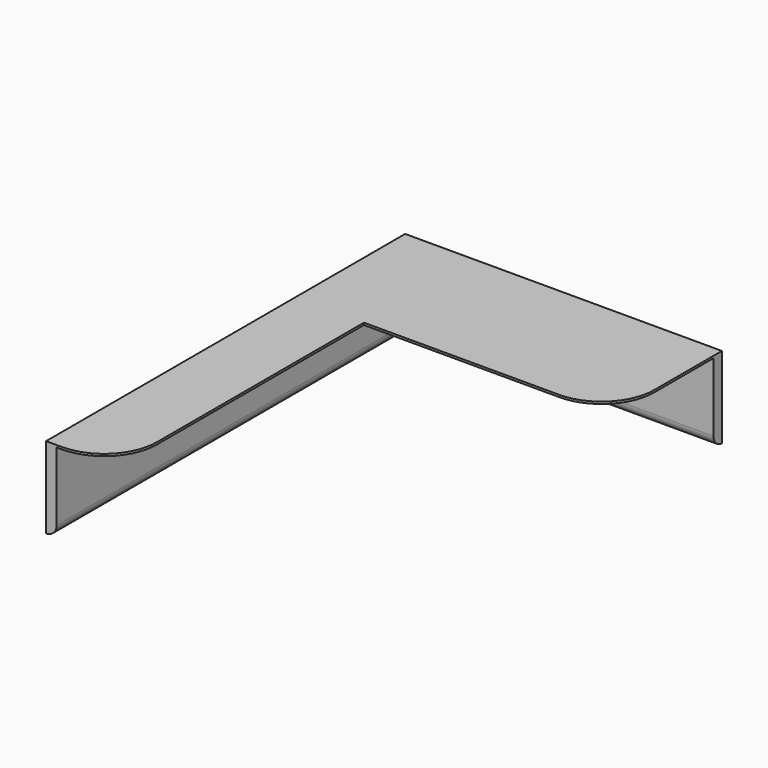
from build123d import *

# Parameters (mm, degrees)
F1_DEPTH = 0.4
F3_DEPTH = 15
F4_R     = 1.99999
F5_R     = 10


# Not quite as in the source:
# - a fillet or chamfer is up to 0.001 mm smaller than in the source, because OpenCascade refuses the exact size


with BuildPart() as f1:
    # F0 (on Top) → F1 (new body)
    with BuildSketch(Plane.XY):
        Polygon((-13, -59), (0, -59), (0, 0), (47, 0), (47, 26), (-13, 26), (-13, 0), align=None)
    extrude(amount=F1_DEPTH)

    # F2 (on face) → F3 (join)
    with BuildSketch(Plane(origin=(0, 0, 0), x_dir=(1, 0, 0), z_dir=(0, 0, -1))):
        Polygon((-13, 59), (-13, -26), (-11, -26), (47, -26), (47, -24), (-11, -24), (-11, 59), align=None)
    extrude(amount=F3_DEPTH)

    # F4 (radius 2 in the source; OpenCascade refuses exactly that, so slightly less here)
    f4_edges = [f1.edges().sort_by_distance(p)[0] for p in [
        (-11, -17.5, -15),
        (18, 24, -15),
    ]]
    fillet(f4_edges, radius=F4_R)

    # F5
    f5_edges = [f1.edges().sort_by_distance(p)[0] for p in [
        (0, -59, 0.2),
        (47, 0, 0.2),
    ]]
    fillet(f5_edges, radius=F5_R)


solid = f1.part
